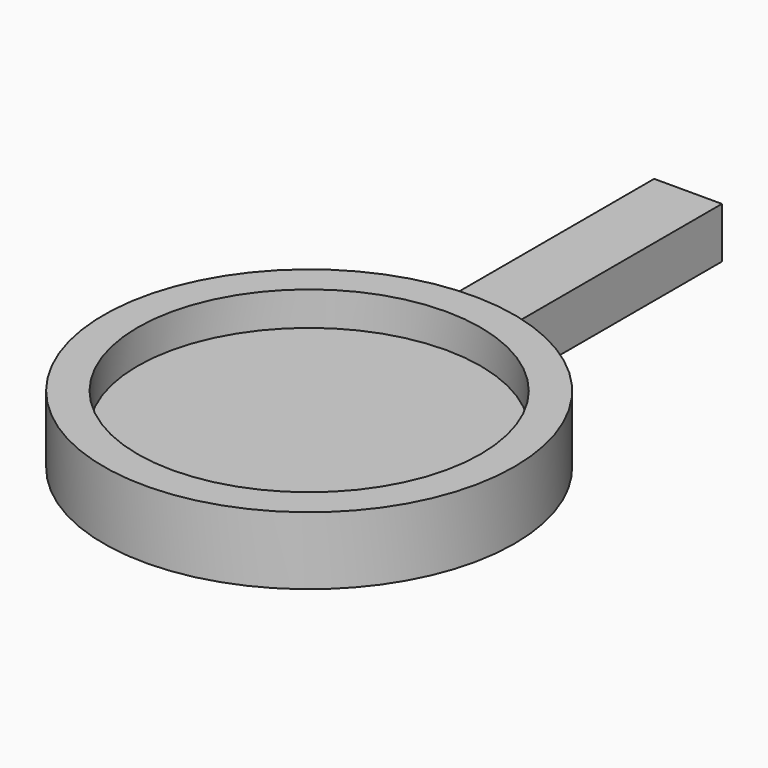
from build123d import *

# Parameters (mm, degrees)
F0_R     = 9.625
F1_DEPTH = 1.5875
F2_R     = 9.625
F2_R_2   = 8.0375
F3_DEPTH = 1.5875
F4_W     = 3.175
F4_H     = 12.7
F5_DEPTH = 2.38125


with BuildPart() as f1:
    # F0 (on Top) → F1 (new body)
    with BuildSketch(Plane.XY):
        Circle(F0_R)
    extrude(amount=F1_DEPTH)

    # F2 (on face) → F3 (join)
    with BuildSketch(Plane.XY.offset(1.5875)):
        Circle(F2_R)
        Circle(F2_R_2, mode=Mode.SUBTRACT)
    extrude(amount=F3_DEPTH)

    # F4 (on Top) → F5 (join)
    with BuildSketch(Plane.XY):
        with Locations((0, 15.8431801179)):
            Rectangle(F4_W, F4_H)
    extrude(amount=F5_DEPTH)


solid = f1.part
